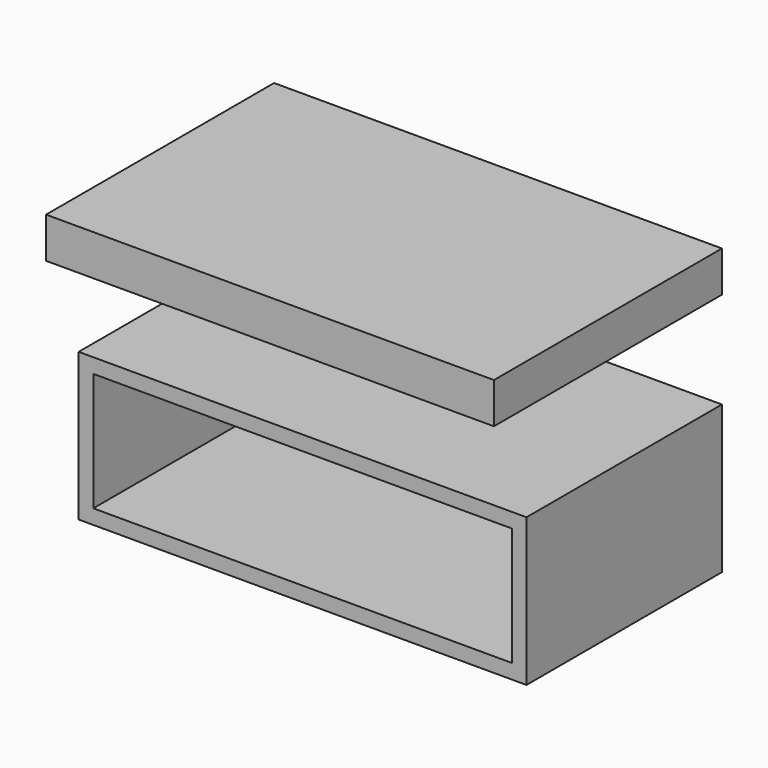
from build123d import *

# Parameters (mm, degrees)
F4_W     = 550
F4_H     = 50
F5_DEPTH = 350
F6_W     = 550
F6_H     = 181.3333858525
F6_W_2   = 514
F6_H_2   = 145.3333858525
F7_DEPTH = 300


# Not quite as in the source:
# - the program builds the solid bodies; features that only make, move or delete a surface that nothing else refers to are left out


with BuildPart() as f5:
    # F4 (on face) → F5 (new body)
    with BuildSketch(Plane(origin=(0, 0, 0), x_dir=(-1, 0, 0), z_dir=(0, 1, 0))):
        with Locations((0, 325)):
            Rectangle(F4_W, F4_H)
    extrude(amount=-F5_DEPTH)


with BuildPart() as f7:
    # F6 (on face) → F7 (new body)
    with BuildSketch(Plane(origin=(0, 0, 0), x_dir=(-1, 0, 0), z_dir=(0, 1, 0))):
        with Locations((0, 90.6666929262)):
            Rectangle(F6_W, F6_H)
        with Locations((0, 90.6666929262)):
            Rectangle(F6_W_2, F6_H_2, mode=Mode.SUBTRACT)
    extrude(amount=-F7_DEPTH)


solid = Compound([f5.part, f7.part])
